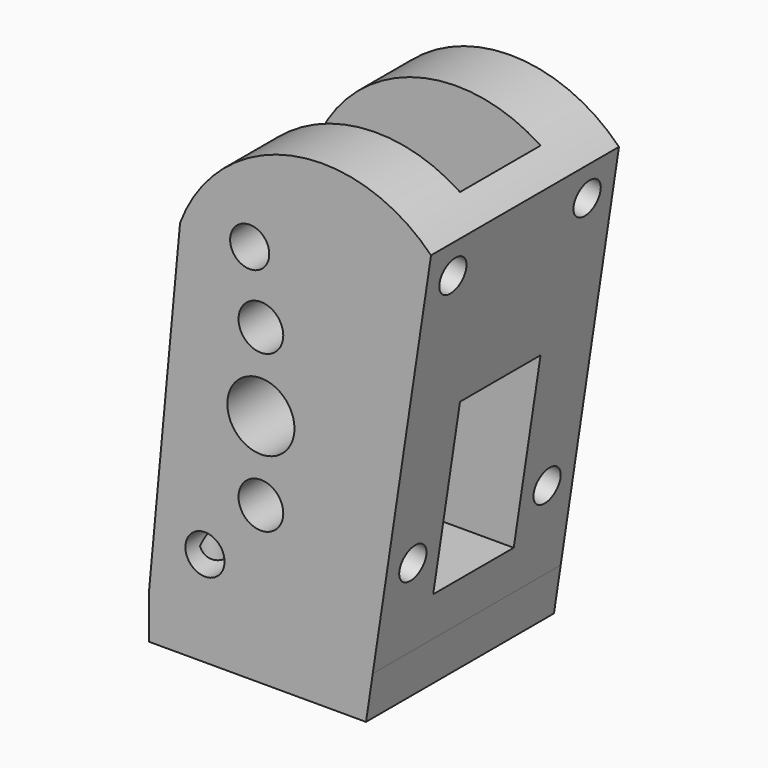
from build123d import *

# Parameters (mm, degrees)
F1_DEPTH    = 10.5
F3_DEPTH    = 4.5
F6_D        = 3.5
F7_T1_DEPTH = 9
F8_R        = 2
F9_DEPTH    = 12.5
F8_R_2      = 3
F11_DEPTH   = 4
F13_DEPTH   = 20
F16_D       = 3
F16_DEPTH   = 8
F16_TIP     = 0.9012909285
F18_D       = 3
F18_DEPTH   = 8
F18_TIP     = 0.9012909285


# Not quite as in the source:
# - a fillet or chamfer that OpenCascade refuses, or shapes differently, is made with other operations: its cross-section is extruded or revolved along the edge and cut away or added


with BuildPart() as f1:
    # F0 (on Front) → F1 (new body, symmetric)
    with BuildSketch(Plane.XZ):
        with BuildLine():
            Line((-10, 0), (10, 0))
            Line((10, 0), (15.209575871, 34.6101187407))
            ThreePointArc((15.209575871, 34.6101187407), (2.6933109979, 38.3883800382), (-7.2260939759, 29.8714821422))
            Line((-7.2260939759, 29.8714821422), (-10, 0))
        make_face()
    extrude(amount=F1_DEPTH, both=True)


with BuildPart() as f3:
    # F2 (on Front) → F3 (new body, symmetric)
    with BuildSketch(Plane.XZ):
        Polygon((-2, 4), (13, 4), (13, 39), (-15, 39), (-15, 0), (-2.371445382, 0), align=None)
    extrude(amount=F3_DEPTH, both=True)


with BuildPart() as f1_1:
    add(f1.part)

    # F4: cut F3
    add(f3.part, mode=Mode.SUBTRACT)

    # F6 (through all)
    with Locations(Plane.XZ.offset(10.5)):
        with Locations((-1, 30), (-5, 4.5)):
            Hole(F6_D / 2)

    # F7: chamfer of 5 on 1 edges, made by hand

    # F7_s2 → F7_t1 (cut)
    with BuildSketch(Plane.XZ.offset(-4.5)):
        Polygon((3, 4), (-2.4623176707, -0.978580357), (-2, 4), align=None)
    extrude(amount=F7_T1_DEPTH, mode=Mode.SUBTRACT)


with BuildPart() as f9:
    # F8 (on Front) → F9 (new body, symmetric)
    with BuildSketch(Plane.XZ):
        with Locations((0, 24)):
            Circle(F8_R)
    extrude(amount=F9_DEPTH, both=True)


with BuildPart() as f9b:
    # F8 (on Front) → F9, piece 2 (new body, symmetric)
    with BuildSketch(Plane.XZ):
        with Locations((0, 17)):
            Circle(F8_R_2)
    extrude(amount=F9_DEPTH, both=True)


with BuildPart() as f9c:
    # F8 (on Front) → F9, piece 3 (new body, symmetric)
    with BuildSketch(Plane.XZ):
        with Locations((0, 10)):
            Circle(F8_R)
    extrude(amount=F9_DEPTH, both=True)


with BuildPart() as f1_2:
    add(f1_1.part)

    # F10: cut F9c, F9b, F9
    add(f9c.part, mode=Mode.SUBTRACT)
    add(f9b.part, mode=Mode.SUBTRACT)
    add(f9.part, mode=Mode.SUBTRACT)

    # F11 (add): a face of the model
    f11_faces = [f1_2.faces().sort_by_distance(p)[0] for p in [
        (1.2885403927, 0, 0),
    ]]
    extrude(f11_faces, amount=F11_DEPTH)


with BuildPart() as f13:
    # F12 (on Front) → F13 (new body, symmetric)
    with BuildSketch(Plane.XZ):
        Polygon((10, -10), (10, 0), (8.4947824334, -10), align=None)
    extrude(amount=F13_DEPTH, both=True)


with BuildPart() as f1_3:
    add(f1_2.part)

    # F14: cut F13
    add(f13.part, mode=Mode.SUBTRACT)

    # F16
    with Locations(Plane(origin=(0, 0, -4), x_dir=(1, 0, 0), z_dir=(0, 0, -1))):
        with Locations((-7, 7.5), (6.3979129734, 7.5), (6.3979129734, -7.5), (-7, -7.5)):
            Hole(F16_D / 2, depth=F16_DEPTH)
            with Locations((0, 0, -(F16_DEPTH + F16_TIP / 2))):  # 118° drill point
                Cone(0, F16_D / 2, F16_TIP, mode=Mode.SUBTRACT)

    # F18
    with Locations(Plane(origin=(9.7784515857, 0, -1.4718697101), x_dir=(0, 1, 0), z_dir=(0.9888605354, 0, -0.1488450249))):
        with Locations((-7.5, 33.4884502488), (7.5, 33.4884502488), (-7.5, 9.4433904486), (7.5, 9.4433904486)):
            Hole(F18_D / 2, depth=F18_DEPTH)
            with Locations((0, 0, -(F18_DEPTH + F18_TIP / 2))):  # 118° drill point
                Cone(0, F18_D / 2, F18_TIP, mode=Mode.SUBTRACT)


solid = f1_3.part
